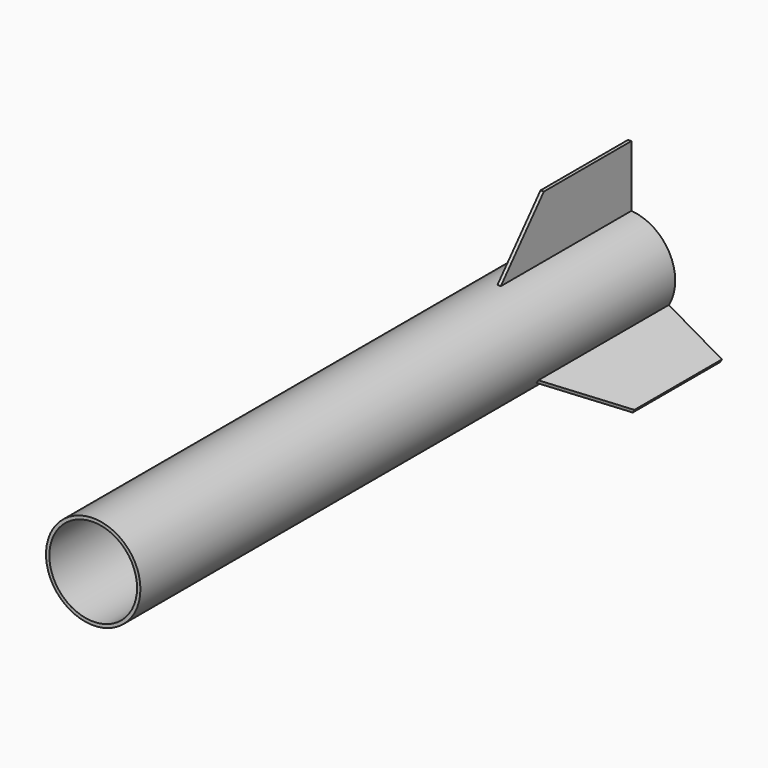
from build123d import *

# Parameters (mm, degrees)
F0_R     = 11.3
F0_R_2   = 10.5
F1_DEPTH = 160
F3_DEPTH = 0.8
F4_COUNT = 3


with BuildPart() as f1:
    # F0 (on Front) → F1 (new body)
    with BuildSketch(Plane.XZ):
        Circle(F0_R)
        Circle(F0_R_2, mode=Mode.SUBTRACT)
    extrude(amount=F1_DEPTH)


with BuildPart() as f3:
    # F2 (on Right) → F3 (new body)
    with BuildSketch(Plane.YZ):
        Polygon((-40, 10.1933907717), (0, 10.1933907717), (0, 25.9597730054), (-26.1820424762, 25.9597730054), align=None)
    extrude(amount=F3_DEPTH)


with BuildPart() as f4_1:
    # F4: instance of F3
    add(f3.part.rotate(Axis((0, 0, 0), (0, 1, 0)), 1 * 360 / F4_COUNT))


with BuildPart() as f4_2:
    # F4: instance of F3
    add(f3.part.rotate(Axis((0, 0, 0), (0, 1, 0)), 2 * 360 / F4_COUNT))


solid = Compound([f1.part, f3.part, f4_1.part, f4_2.part])
